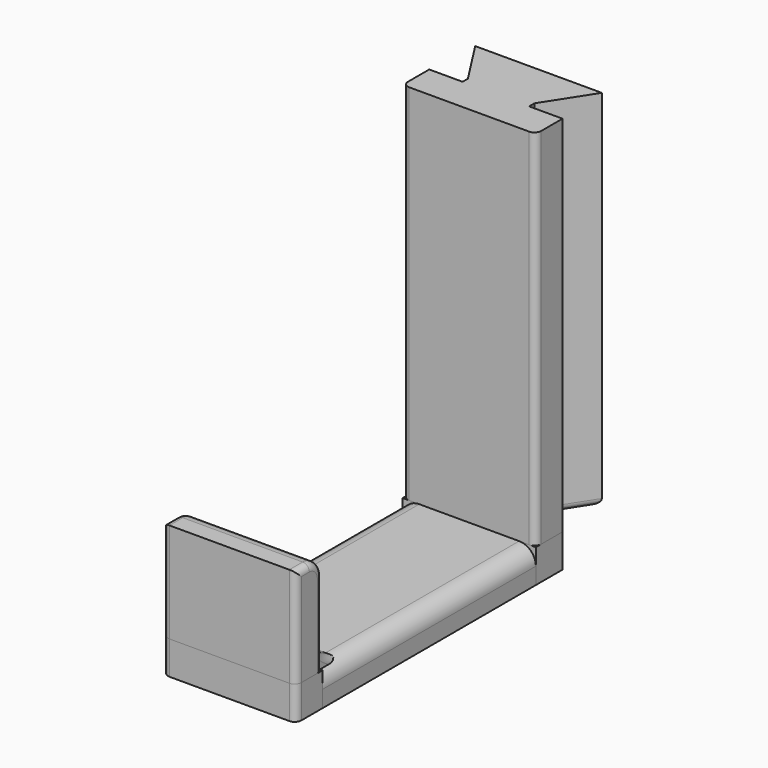
from build123d import *

# Parameters (mm, degrees)
F1_START = 5
F0_W     = 10
F0_H     = 1
F1_DEPTH = 54.6
F2_START = 5
F2_DEPTH = 54.6
F3_START = 5
F0_W_2   = 20
F0_H_2   = 5
F3_DEPTH = 15
F0_H_3   = 40
F4_DEPTH = 5
F5_DEPTH = 5
F6_R     = 2.5
F6_2_R   = 2.5
F8_START = 1
F8_DEPTH = 18
F9_R     = 1
F9_2_R   = 1
F9_3_R   = 1
F9_4_R   = 1


# Not quite as in the source:
# - two fillets or chamfers of one size are made in one step
# - a feature names something its author has since deleted; it is built from what else it names


with BuildPart() as f1:
    # F0 (on Top) → F1 (new body)
    with BuildSketch(Plane.XY.offset(F1_START)):
        Polygon((0.5, 58), (5, 51), (15, 51), (19.5, 58), align=None)
        with Locations((10, 50.5)):
            Rectangle(F0_W, F0_H)
        Polygon((0, 50), (0, 45), (20, 45), (20, 50), (15, 50), (5, 50), align=None)
    extrude(amount=F1_DEPTH)

    # F0 (on Top) → F2 (join)
    with BuildSketch(Plane.XY.offset(F2_START)):
        Polygon((0, 50), (0, 45), (20, 45), (20, 50), (15, 50), (5, 50), align=None)
    extrude(amount=F2_DEPTH)

    # F9
    f9_edges = [f1.edges().sort_by_distance(p)[0] for p in [
        (0, 45, 32.3),
        (20, 45, 32.3),
        (2.75, 54.5, 5),
        (10, 58, 5),
        (5, 50.5, 5),
        (15, 50.5, 5),
        (17.25, 54.5, 5),
    ]]
    fillet(f9_edges, radius=F9_R)


with BuildPart() as f3:
    # F0 (on Top) → F3 (new body)
    with BuildSketch(Plane.XY.offset(F3_START)):
        with Locations((10, 2.5)):
            Rectangle(F0_W_2, F0_H_2)
    extrude(amount=F3_DEPTH)

    # F6
    f6_edges = [f3.edges().sort_by_distance(p)[0] for p in [
        (10, 5, 20),
    ]]
    fillet(f6_edges, radius=F6_R)

    # F9#2
    f9_2_edges = [f3.edges().sort_by_distance(p)[0] for p in [
        (20, 5, 11.25),
        (0, 5, 11.25),
        (0, 0, 12.5),
        (20, 0, 12.5),
        (0, 4.267767, 19.267767),
        (0, 1.25, 20),
        (20, 4.267767, 19.267767),
        (20, 1.25, 20),
    ]]
    fillet(f9_2_edges, radius=F9_2_R)


with BuildPart() as f4:
    # F0 (on Top) → F4 (new body)
    with BuildSketch(Plane.XY):
        with Locations((10, 25)):
            Rectangle(F0_W_2, F0_H_3)
    extrude(amount=F4_DEPTH)

    # F6#2
    f6_2_edges = [f4.edges().sort_by_distance(p)[0] for p in [
        (20, 25, 5),
        (0, 25, 5),
    ]]
    fillet(f6_2_edges, radius=F6_2_R)


with BuildPart() as f5:
    # F0 (on Top) → F5 (new body)
    with BuildSketch(Plane.XY):
        with Locations((10, 2.5)):
            Rectangle(F0_W_2, F0_H_2)
    extrude(amount=F5_DEPTH)

    # F9#3
    f9_3_edges = [f5.edges().sort_by_distance(p)[0] for p in [
        (20, 0, 2.5),
        (0, 0, 2.5),
    ]]
    fillet(f9_3_edges, radius=F9_3_R)


with BuildPart() as f5b:
    # F0 (on Top) → F5, piece 2 (new body)
    with BuildSketch(Plane.XY):
        Polygon((0, 50), (0, 45), (20, 45), (20, 50), (15, 50), (5, 50), align=None)
    extrude(amount=F5_DEPTH)


with BuildPart() as f8:
    # F7 (on Right) → F8 (new body)
    with BuildSketch(Plane.YZ.offset(F8_START)):
        with BuildLine():
            Line((4.6167019755, 4.4840211049), (9.9377890915, 4.4840211049))
            add(Edge.make_bspline(
                [(4.2957553071, 12.42066134), (4.6167019755, 10.3172202345), (5.2240094479, 6.3370091055), (8.4273385535, 5.0777796032), (9.9377890915, 4.4840211049)],
                knots=[0, 0, 0, 0, 0.5284747561, 1, 1, 1, 1], degree=3))
            Line((4.2957553071, 12.42066134), (4.6167019755, 4.4840211049))
        make_face()
    extrude(amount=F8_DEPTH)

    # F9#4
    f9_4_edges = [f8.edges().sort_by_distance(p)[0] for p in [
        (1, 5.651637, 7.360722),
        (19, 5.651637, 7.360722),
    ]]
    fillet(f9_4_edges, radius=F9_4_R)


solid = Compound([f1.part, f3.part, f4.part, f5.part, f5b.part, f8.part])
